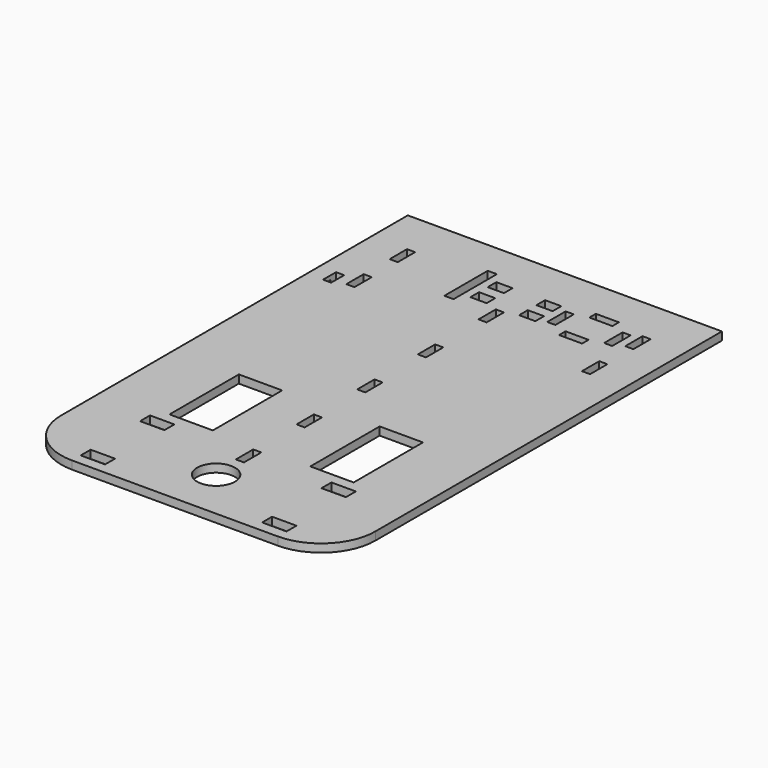
from build123d import *

# Parameters (mm, degrees)
F0_W      = 57.15
F0_H      = 29.21
F0_R      = 44.45
F1_DEPTH  = 19.05
F2_W      = 19.05
F2_H      = 50.8
F3_DEPTH  = 25.4
F4_W      = 19.05
F4_H      = 50.8
F5_DEPTH  = 25.4
F6_W      = 38.1
F6_H      = 25.4
F6_W_2    = 53.975
F6_H_2    = 19.05
F6_W_3    = 19.05
F6_H_3    = 53.975
F7_DEPTH  = 25.4
F8_R      = 127
F10_DEPTH = 25.4
F11_W     = 6.35
F11_H     = 6.35
F12_DEPTH = 9.525


# Not quite as in the source:
# - a feature names something its author has since deleted; it is built from what else it names


with BuildPart() as f1:
    # F0 (on Top) → F1 (new body)
    with BuildSketch(Plane.XY):
        Polygon((358.775, 0), (0, 0), (0, -889), (152.4, -889), (152.4, -685.8), (254, -685.8), (254, -889), (482.6, -889), (482.6, -685.8), (584.2, -685.8), (584.2, -889), (736.6, -889), (736.6, 0), (377.825, 0), align=None)
        Polygon((152.4, -889), (0, -889), (0, -1143), (358.775, -1143), (377.825, -1143), (736.6, -1143), (736.6, -889), (584.2, -889), (482.6, -889), (254, -889), align=None)
        with Locations((155.575, -1102.995)):
            Rectangle(F0_W, F0_H, mode=Mode.SUBTRACT)
        with Locations((155.575, -929.005)):
            Rectangle(F0_W, F0_H, mode=Mode.SUBTRACT)
        with Locations((368.3, -1022.35)):
            Circle(F0_R, mode=Mode.SUBTRACT)
        with Locations((581.025, -1102.995)):
            Rectangle(F0_W, F0_H, mode=Mode.SUBTRACT)
        with Locations((581.025, -929.005)):
            Rectangle(F0_W, F0_H, mode=Mode.SUBTRACT)
    extrude(amount=F1_DEPTH)

    # F2 (on face) → F3 (cut)
    with BuildSketch(Plane.XY.offset(19.05)):
        with Locations((368.3, -215.9)):
            Rectangle(F2_W, F2_H)
        with Locations((368.3, -393.7)):
            Rectangle(F2_W, F2_H)
        with Locations((368.3, -571.5)):
            Rectangle(F2_W, F2_H)
        with Locations((368.3, -749.3)):
            Rectangle(F2_W, F2_H)
        with Locations((368.3, -927.1)):
            Rectangle(F2_W, F2_H)
    extrude(amount=-F3_DEPTH, mode=Mode.SUBTRACT)

    # F4 (on face) → F5 (cut)
    with BuildSketch(Plane.XY.offset(19.05)):
        with Locations((92.075, -130.9968532642)):
            Rectangle(F4_W, F4_H)
        with Locations((92.075, -257.9968532642)):
            Rectangle(F4_W, F4_H)
        with Locations((644.525, -130.9968532642)):
            Rectangle(F4_W, F4_H)
        with Locations((644.525, -257.9968532642)):
            Rectangle(F4_W, F4_H)
    extrude(amount=-F5_DEPTH, mode=Mode.SUBTRACT)

    # F6 (on face) → F7 (cut)
    with BuildSketch(Plane.XY.offset(19.05)):
        with Locations((311.15, -118.2968532642)):
            Rectangle(F6_W, F6_H)
        with Locations((311.15, -169.0968532642)):
            Rectangle(F6_W, F6_H)
        Polygon((444.5, -170.6843532642), (444.5, -156.3968532642), (406.4, -156.3968532642), (406.4, -181.7968532642), (444.5, -181.7968532642), align=None)
        Polygon((444.5, -116.7093532642), (444.5, -105.5968532642), (406.4, -105.5968532642), (406.4, -130.9968532642), (444.5, -130.9968532642), align=None)
        with Locations((539.75, -99.2468532642)):
            Rectangle(F6_W_2, F6_H_2)
        with Locations((473.075, -143.6968532642)):
            Rectangle(F6_W_3, F6_H_3)
        with Locations((539.75, -188.1468532642)):
            Rectangle(F6_W_2, F6_H_2)
        with Locations((606.425, -143.6968532642)):
            Rectangle(F6_W_3, F6_H_3)
        Polygon((273.05, -207.1968532642), (273.05, -143.6968532642), (273.05, -80.1968532642), (251.5147030354, -80.1968532642), (251.5147030354, -207.1968532642), align=None)
    extrude(amount=-F7_DEPTH, mode=Mode.SUBTRACT)

    # F8
    f8_edges = [f1.edges().sort_by_distance(p)[0] for p in [
        (0, -1143, 9.525),
        (736.6, -1143, 9.525),
    ]]
    fillet(f8_edges, radius=F8_R)

    # F9 (on face) → F10 (cut)
    with BuildSketch(Plane.XY.offset(19.05)):
        Polygon((57.15, -257.9968532642), (38.1, -257.9968532642), (38.1, -273.8015651703), (38.1, -280.3961336613), (38.1, -296.0968532642), (57.15, -296.0968532642), (57.15, -280.3961336613), (57.15, -273.8015651703), align=None)
    extrude(amount=-F10_DEPTH, mode=Mode.SUBTRACT)

    # F11 (on face) → F12 (cut)
    with BuildSketch(Plane(origin=(0, 0, 0), x_dir=(1, 0, 0), z_dir=(0, 0, -1))):
        with Locations((34.925, 277.0468532642)):
            Rectangle(F11_W, F11_H)
        with Locations((60.325, 277.0468532642)):
            Rectangle(F11_W, F11_H)
    extrude(amount=-F12_DEPTH, mode=Mode.SUBTRACT)


solid = f1.part
